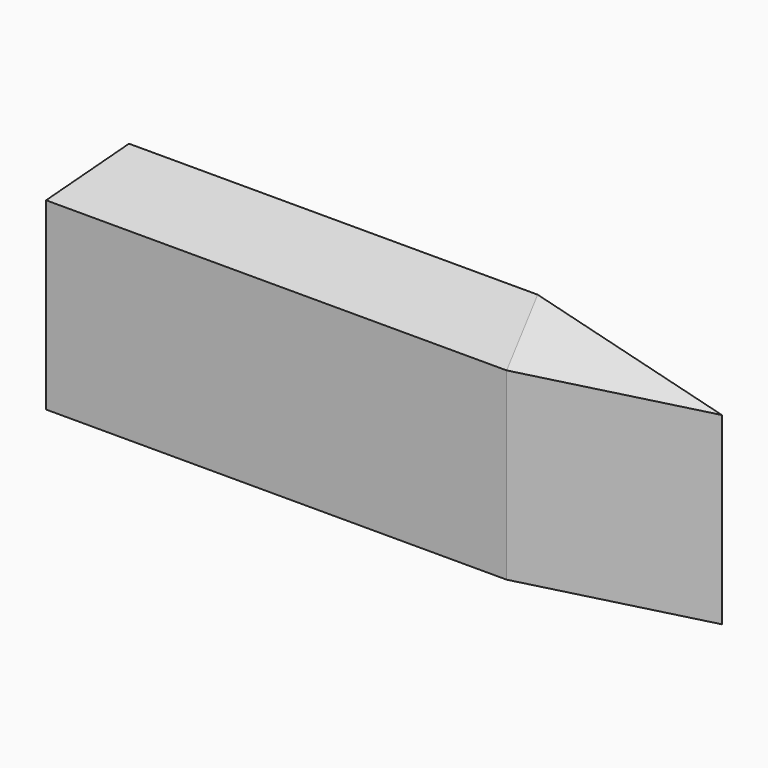
from build123d import *

# Parameters (mm, degrees)
F0_W     = 50
F0_H     = 10
F1_DEPTH = 25
F2_SIZE  = 4.99999


# Not quite as in the source:
# - a fillet or chamfer is up to 0.001 mm smaller than in the source, because OpenCascade refuses the exact size


with BuildPart() as f1:
    # F0 (on Top) → F1 (new body)
    with BuildSketch(Plane.XY):
        with Locations((-24.5698342215, 0)):
            Rectangle(F0_W, F0_H)
        Polygon((0.4301657785, 5), (0.4301657785, -5), (19.7950825095, 0), align=None)
    extrude(amount=F1_DEPTH)

    # F2 (size 5 in the source; OpenCascade refuses exactly that, so slightly less here)
    f2_edges = [f1.edges().sort_by_distance(p)[0] for p in [
        (-24.569834, -5, 25),
        (-49.569834, 0, 25),
        (-24.569834, 5, 25),
        (10.112624, 2.5, 25),
        (10.112624, -2.5, 25),
    ]]
    chamfer(f2_edges, length=F2_SIZE)


solid = f1.part
